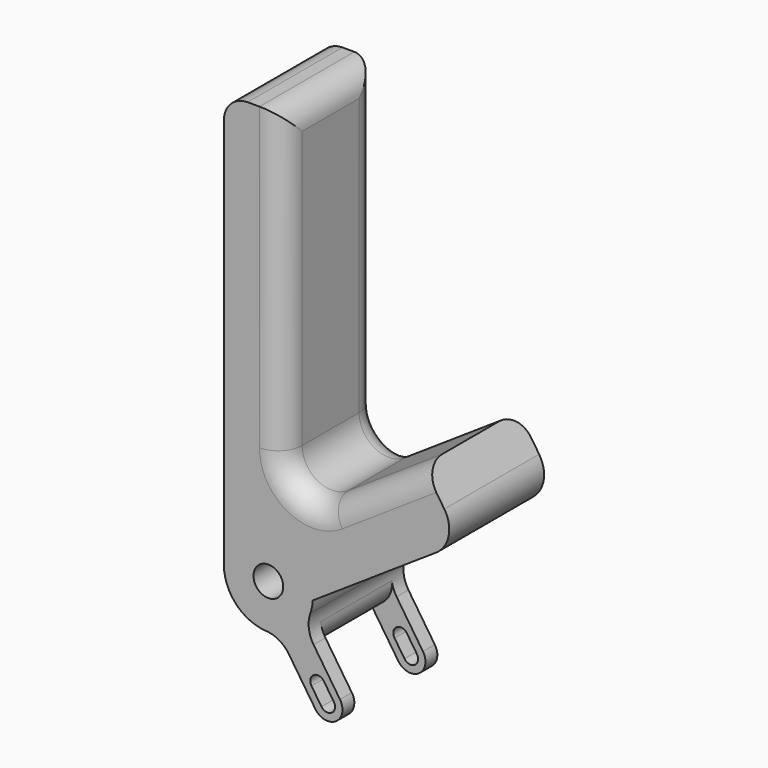
from build123d import *

# Parameters (mm, degrees)
F0_R        = 3.175
F1_DEPTH    = 25.4
F2_R        = 5.08
F3_W        = 19.05
F3_H        = 15.7622399921
F4_DEPTH    = 6.35
F5_T1_DEPTH = 19.05


# Not quite as in the source:
# - a fillet or chamfer that OpenCascade refuses, or shapes differently, is made with other operations: its cross-section is extruded or revolved along the edge and cut away or added


with BuildPart() as f1:
    # F0 (on Front) → F1 (new body)
    with BuildSketch(Plane.XZ):
        with BuildLine():
            ThreePointArc((-0.6915815922, -12.1052896192), (-1.7090267403, -9.3705639378), (-1.3960508414, -6.4695356255))
            ThreePointArc((-1.3960508414, -6.4695356255), (-1.0364150689, -5.1594737521), (-0.8668126136, -3.8115735302))
            Line((-0.8668126136, -3.8115735302), (25.5427133598, 13.7947321605))
            ThreePointArc((25.5427133598, 13.7947321605), (28.2470591636, 17.8329108842), (27.3038968609, 22.6005956999))
            Line((27.3038968609, 22.6005956999), (22.778728087, 29.3883661936))
            Line((22.778728087, 29.3883661936), (2.6693062503, 15.9821192025))
            ThreePointArc((2.6693062503, 15.9821192025), (-3.8493348951, 15.6670107863), (-7.2030337688, 21.2656427228))
            Line((-7.2030337688, 21.2656427228), (-7.2030337688, 85.6005759959))
            Line((-7.2030337688, 85.6005759959), (-19.9030337688, 85.6005759959))
            Line((-19.9030337688, 85.6005759959), (-19.9030337688, -3.2994240041))
            ThreePointArc((-19.9030337688, -3.2994240041), (-17.2975054683, -9.8451505795), (-10.9063857057, -12.8097588684))
            ThreePointArc((-10.9063857057, -12.8097588684), (-8.1081380718, -13.6366381587), (-5.9751009613, -15.6276358652))
            Line((-5.9751009613, -15.6276358652), (-0.3197934533, -24.1105971271))
            ThreePointArc((-0.3197934533, -24.1105971271), (4.0831393542, -24.9911836886), (4.9637259157, -20.5882508811))
            Line((4.9637259157, -20.5882508811), (-0.6915815922, -12.1052896192))
        make_face()
        with Locations((-10.3780337688, -3.2994240041)):
            Circle(F0_R, mode=Mode.SUBTRACT)
        with BuildLine():
            ThreePointArc((3.6428460735, -21.4688374426), (3.2025527927, -23.6703038464), (1.0010863889, -23.2300105656))
            Line((1.0010863889, -23.2300105656), (-1.131874873, -20.0305686727))
            ThreePointArc((-1.131874873, -20.0305686727), (-0.6915815922, -17.829102269), (1.5098848115, -18.2693955497))
            Line((1.5098848115, -18.2693955497), (3.6428460735, -21.4688374426))
        make_face(mode=Mode.SUBTRACT)
    extrude(amount=F1_DEPTH)

    # F2
    f2_edges = [f1.edges().sort_by_distance(p)[0] for p in [
        (-7.203034, -25.4, 53.433109),
        (-7.203034, 0, 53.433109),
        (-7.203034, -12.7, 85.600576),
        (-19.903034, -12.7, 85.600576),
    ]]
    fillet(f2_edges, radius=F2_R)

    # F3 (on face) → F4 (cut, through all)
    with BuildSketch(Plane(origin=(-6.0658440035, 0, -4.0438960023), x_dir=(0, 1, 0), z_dir=(0.8320502943, 0, 0.5547001962))):
        with Locations((-12.7, -17.5697093418)):
            Rectangle(F3_W, F3_H)
    extrude(amount=-F4_DEPTH, mode=Mode.SUBTRACT)

    # F5: fillet of radius 5.08 on 6 edges, made by hand

    # F5_s2 → F5_t1 (cut)
    with BuildSketch(Plane.XZ.offset(3.175)):
        with BuildLine():
            ThreePointArc((-1.706559996, -9.3900529107), (-2.1228958796, -12.1426914098), (-3.9274812175, -14.262556036))
            Line((-3.9274812175, -14.262556036), (-0.6915815922, -12.1052896192))
            ThreePointArc((-0.6915815922, -12.1052896192), (-1.3560793604, -10.8063623925), (-1.706559996, -9.3900529107))
        make_face()
        with BuildLine():
            ThreePointArc((-8.0910969984, -13.6464109123), (-5.3900707363, -14.3208079809), (-2.739201336, -13.4703694484))
            Line((-2.739201336, -13.4703694484), (-5.9751009613, -15.6276358652))
            ThreePointArc((-5.9751009613, -15.6276358652), (-6.9185346443, -14.5146659151), (-8.0910969984, -13.6464109123))
        make_face()
    extrude(amount=F5_T1_DEPTH, mode=Mode.SUBTRACT)


solid = f1.part
